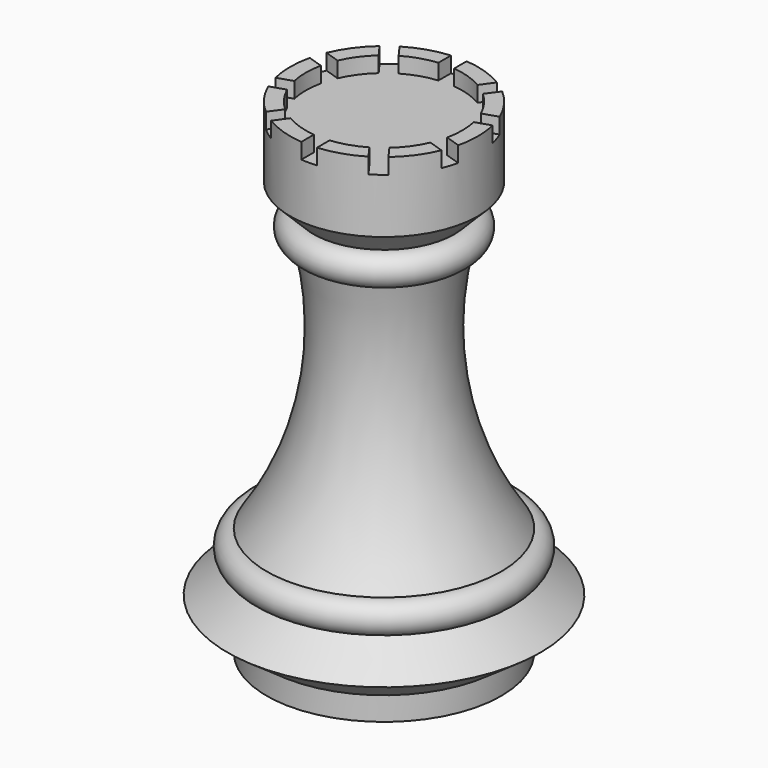
from build123d import *

# Parameters (mm, degrees)
F2_W            = 2.54
F2_H            = 2.54
F3_DEPTH        = 25.401
F3_DEPTH_BACK   = 25.4
F3_COPIES_COUNT = 5
F3_COPIES_ANGLE = 144


# Not quite as in the source:
# - a pattern or mirror of a feature is missing from the dataset's text; its kind, count and spacing are read off the source's solid


with BuildPart() as f1:
    # F0 (on Front) → F1 (revolve)
    with BuildSketch(Plane.XZ):
        with BuildLine():
            Line((0, 76.2), (0, 0))
            Line((0, 0), (19.05, 0))
            Line((19.05, 0), (19.05, 3.81))
            Line((19.05, 3.81), (25.4, 8.255))
            Line((25.4, 8.255), (19.05, 12.7))
            ThreePointArc((19.05, 12.7), (21.59, 15.24), (19.05, 17.78))
            ThreePointArc((19.05, 17.78), (10.9181319171, 37.2896497345), (11.43, 58.42))
            ThreePointArc((11.43, 58.42), (13.97, 60.96), (11.43, 63.5))
            Line((11.43, 63.5), (15.24, 67.31))
            Line((15.24, 67.31), (15.24, 78.74))
            Line((15.24, 78.74), (12.7, 78.74))
            Line((12.7, 78.74), (12.7, 76.2))
            Line((12.7, 76.2), (0, 76.2))
        make_face()
    revolve(axis=Axis((0, 0, 38.1), (0, 0, 1)))

    # F2 (on Front) → F3 (cut, two sides)
    with BuildSketch(Plane.XZ) as f3_sk:
        with Locations((0, 77.47)):
            Rectangle(F2_W, F2_H)
    f3 = extrude(amount=-F3_DEPTH, mode=Mode.SUBTRACT) + extrude(f3_sk.sketch, amount=F3_DEPTH_BACK, mode=Mode.SUBTRACT)

    # F3_copies: F3 ×5 about axis
    f3_copies_axis = Axis((0, 0, 0), (0, 0, 1))
    for i in range(1, F3_COPIES_COUNT):
        add(f3.rotate(f3_copies_axis, i * F3_COPIES_ANGLE / (F3_COPIES_COUNT - 1)), mode=Mode.SUBTRACT)


solid = f1.part
